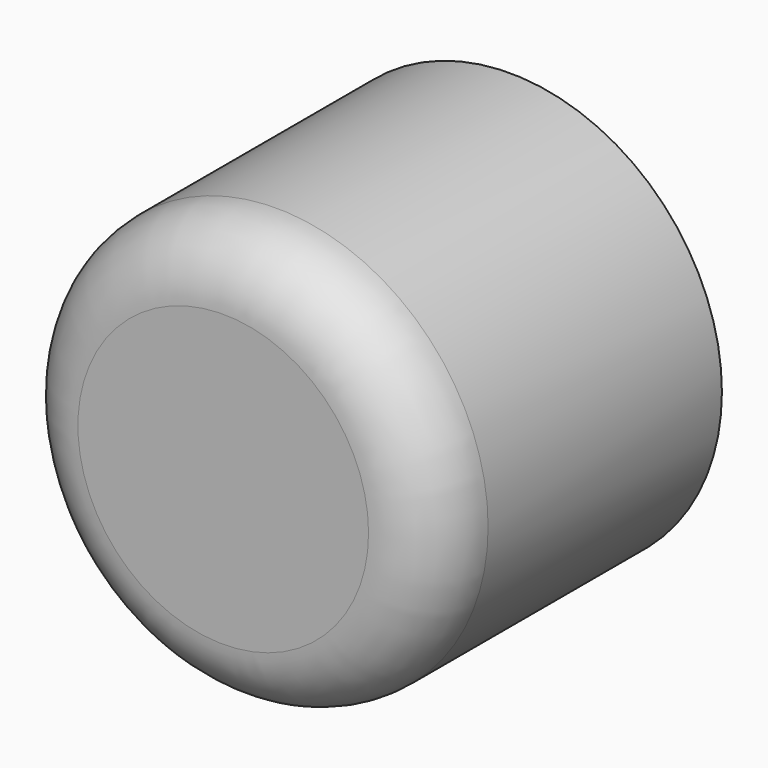
from build123d import *

# Parameters (mm, degrees)
F0_R     = 15.9407183273
F2_DEPTH = 12
F1_R     = 14
F3_DEPTH = 53
F4_DEPTH = 15
F5_R     = 14.3229491525
F6_DEPTH = 25
F7_R     = 5
F8_R     = 4.9147347868
F9_DEPTH = 15.9417183273


# Not quite as in the source:
# - an extrude ends at something that could not be found from the text; its depth is read off the source's solid


with BuildPart() as f2:
    # F0 (on Front) → F2 (new body)
    with BuildSketch(Plane.XZ):
        Circle(F0_R)
    extrude(amount=F2_DEPTH)

    # F1 (on face) → F3 (cut, through all)
    with BuildSketch(Plane.XZ):
        Circle(F1_R)
    extrude(amount=-F3_DEPTH, mode=Mode.SUBTRACT)

    # F4 (add): a face of the model
    f4_faces = [f2.faces().sort_by_distance(p)[0] for p in [
        (0, 0, 0),
    ]]
    extrude(f4_faces, amount=F4_DEPTH)

    # F5 (on face) → F6 (cut)
    with BuildSketch(Plane(origin=(0, 15, 0), x_dir=(-1, 0, 0), z_dir=(0, 1, 0))):
        Circle(F5_R)
    extrude(amount=-F6_DEPTH, mode=Mode.SUBTRACT)

    # F7
    f7_edges = [f2.edges().sort_by_distance(p)[0] for p in [
        (-15.940718, -12, 0),
    ]]
    fillet(f7_edges, radius=F7_R)

    # F8 (on Right) → F9 (cut, through all)
    with BuildSketch(Plane.YZ):
        with Locations((0.8949990151, 0)):
            Circle(F8_R)
    extrude(amount=-F9_DEPTH, mode=Mode.SUBTRACT)


solid = f2.part
